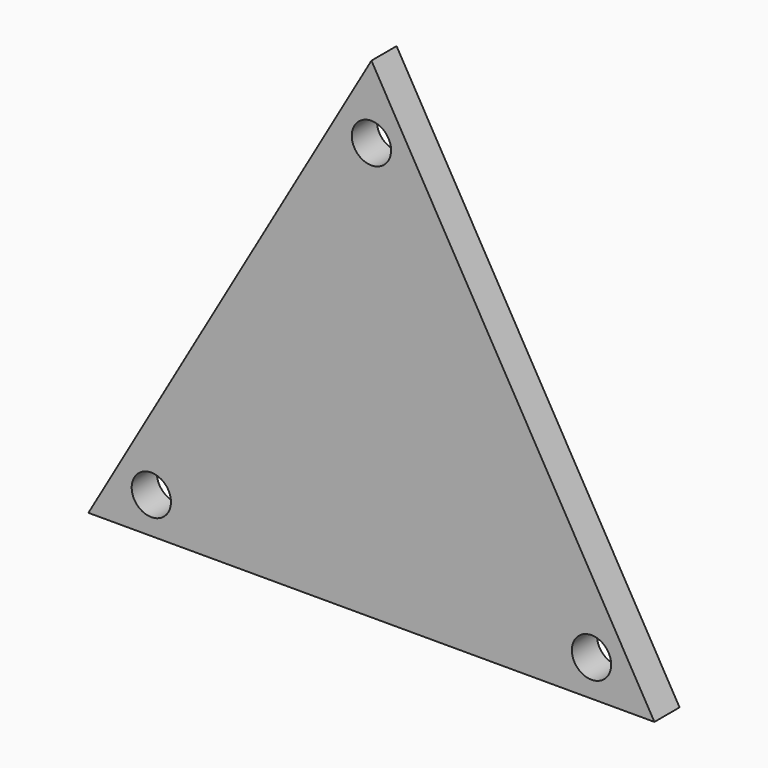
from build123d import *

# Parameters (mm, degrees)
F1_DEPTH = 12.7
F3_D     = 15.875


# Not quite as in the source:
# - a length typed as a fraction of an inch, garbled in the dataset ("3 / 203.2 mm" for 3/8 in), is restored


with BuildPart() as f1:
    # F0 (on Front) → F1 (new body)
    with BuildSketch(Plane.XZ):
        Polygon((114.3, 0), (0, 197.9734073051), (-114.3, 0), align=None)
    extrude(amount=F1_DEPTH)

    # F3 (through all)
    with Locations(Plane.XZ.offset(12.7)):
        with Locations((0, 168.6440136303), (-88.9, 14.6646968374), (88.9, 14.6646968374)):
            Hole(F3_D / 2)


solid = f1.part
